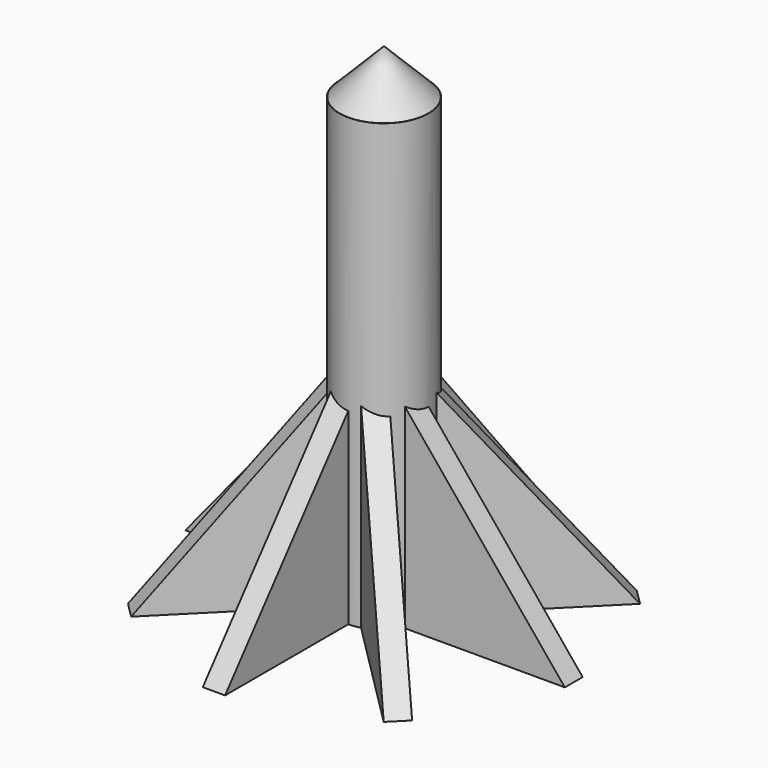
from build123d import *

# Parameters (mm, degrees)
F0_R            = 100
F1_DEPTH        = 1000
F3_DEPTH        = 50
F3_COPIES_COUNT = 8


# Not quite as in the source:
# - a pattern or mirror of a feature is missing from the dataset's text; its kind, count and spacing are read off the source's solid


with BuildPart() as f1:
    # F0 (on Top) → F1 (new body)
    with BuildSketch(Plane.XY):
        Circle(F0_R)
    extrude(amount=F1_DEPTH)

    # F2 (on Right) → F3 (join)
    with BuildSketch(Plane.YZ):
        Polygon((0, 543.3371663094), (0, 0), (445.3816711903, 0), align=None)
    f3 = extrude(amount=F3_DEPTH)

    # F3_copies: F3 ×8 about axis
    f3_copies_axis = Axis((0, 0, 0), (0, 0, 1))
    for i in range(1, F3_COPIES_COUNT):
        add(f3.rotate(f3_copies_axis, i * 360 / F3_COPIES_COUNT))


with BuildPart() as f5:
    # F4 (on Front) → F5 (revolve)
    with BuildSketch(Plane.XZ):
        Polygon((0, 1100.4860401154), (-99.4548052549, 1000.0003576279), (0, 1000.6748437881), align=None)
    revolve(axis=Axis((0, 0, 1000), (0, 0, 1)))


solid = Compound([f1.part, f5.part])
